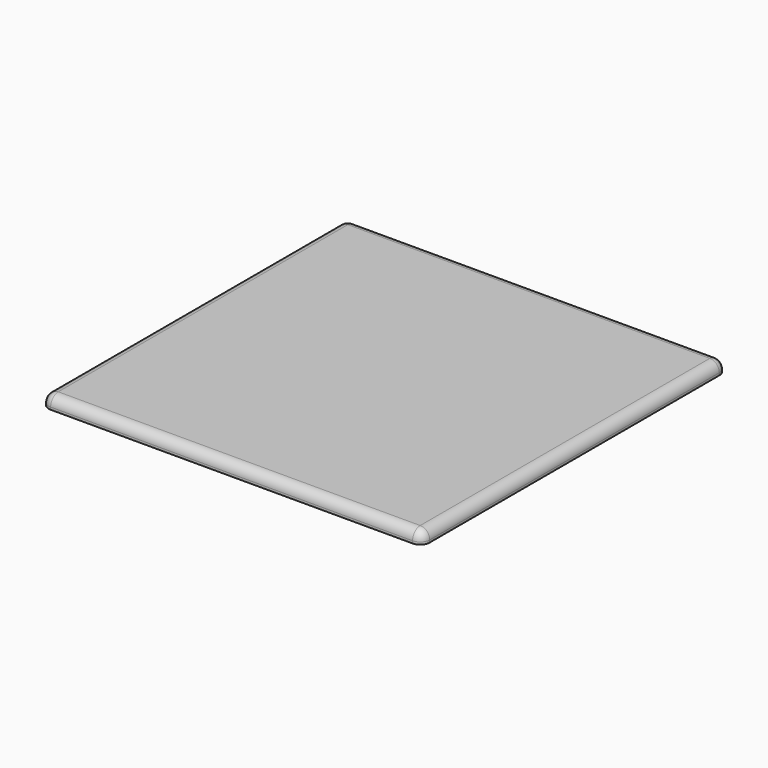
from build123d import *

# Parameters (mm, degrees)
F0_W     = 508
F0_H     = 508
F1_DEPTH = 15.875
F4_R     = 12.7
F5_R     = 12.7
F6_R     = 12.7


# Not quite as in the source:
# - the program builds the solid bodies; features that only make, move or delete a surface that nothing else refers to are left out


with BuildPart() as f1:
    # F0 (on Top) → F1 (new body)
    with BuildSketch(Plane.XY):
        with Locations((-1.661028713, -10.90797159)):
            Rectangle(F0_W, F0_H)
    extrude(amount=F1_DEPTH)

    # F4
    f4_edges = [f1.edges().sort_by_distance(p)[0] for p in [
        (252.338971, 243.092028, 7.9375),
        (252.338971, -264.907972, 7.9375),
    ]]
    fillet(f4_edges, radius=F4_R)

    # F5
    f5_edges = [f1.edges().sort_by_distance(p)[0] for p in [
        (-255.661029, 243.092028, 7.9375),
        (-255.661029, -264.907972, 7.9375),
    ]]
    fillet(f5_edges, radius=F5_R)

    # F6
    f6_edges = [f1.edges().sort_by_distance(p)[0] for p in [
        (-1.661029, 243.092028, 15.875),
        (-251.941285, 239.372285, 15.875),
        (248.619227, 239.372285, 15.875),
        (-255.661029, -10.907972, 15.875),
        (252.338971, -10.907972, 15.875),
        (-251.941285, -261.188228, 15.875),
        (248.619227, -261.188228, 15.875),
        (-1.661029, -264.907972, 15.875),
    ]]
    fillet(f6_edges, radius=F6_R)


solid = f1.part
